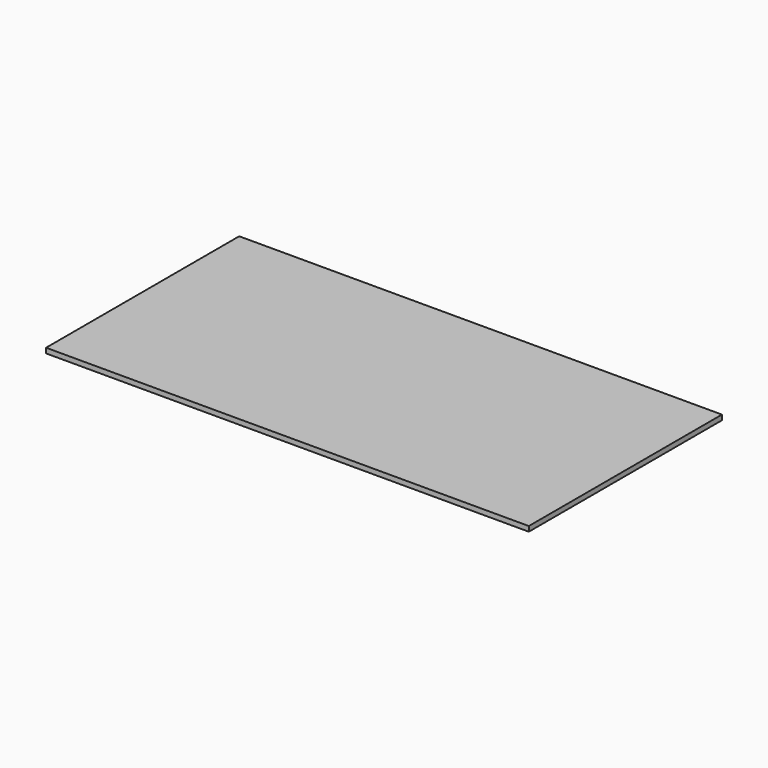
from build123d import *

# Parameters (mm, degrees)
F0_W     = 152.4
F0_H     = 76.2
F1_DEPTH = 1.5875


# Not quite as in the source:
# - a length typed as a fraction of an inch, garbled in the dataset ("3 / 203.2 mm" for 3/8 in), is restored


with BuildPart() as f1:
    # F0 (on Top) → F1 (new body)
    with BuildSketch(Plane.XY):
        Rectangle(F0_W, F0_H)
    extrude(amount=F1_DEPTH)


solid = f1.part
